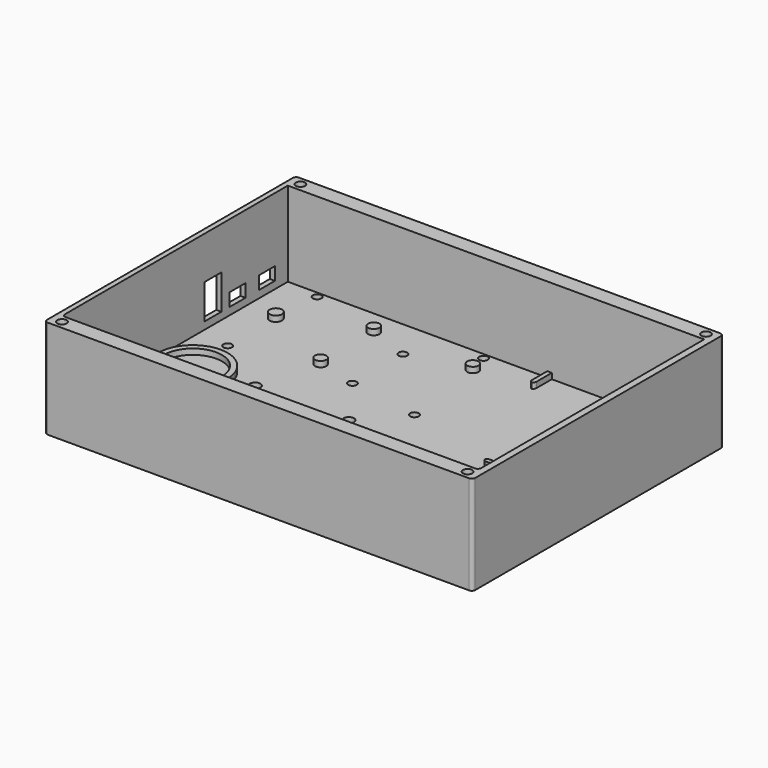
from build123d import *

# Parameters (mm, degrees)
F5_W         = 192.786
F5_H         = 141.3764
F7_DEPTH     = 44.45
F12_W        = 187.452
F12_H        = 127
F14_DEPTH    = 38.1
F4_R         = 15.621
F4_R_2       = 13.081
F13_W        = 2.032
F13_H        = 10.16
F13_W_2      = 10.16
F13_H_2      = 2.032
F15_DEPTH    = 8.89
F16_DEPTH    = 2.9972
F17_DEPTH    = 3.81
F10_R        = 2.3749
F18_DEPTH    = 25.4
F3_R         = 1.9304
F19_DEPTH    = 25.4
F11_R        = 2.54
F11_R_2      = 2.794
F20_DEPTH    = 8.89
F21_W        = 8.89
F21_H        = 5.842
F21_W_2      = 9.525
F21_H_2      = 15.621
F22_DEPTH    = 25.4
F23_R        = 2.0828
F24_DEPTH    = 4.318
F25_T1_DEPTH = 41.91
F25_T3_DEPTH = 52.07
F25_T5_DEPTH = 6.35


# Not quite as in the source:
# - a fillet or chamfer that OpenCascade refuses, or shapes differently, is made with other operations: its cross-section is extruded or revolved along the edge and cut away or added


with BuildPart() as f7:
    # F5 (on Top) → F7 (new body)
    with BuildSketch(Plane.XY):
        with Locations((-4.773771323, -23.1295908162)):
            Rectangle(F5_W, F5_H)
    extrude(amount=F7_DEPTH)

    # F12 (on face) → F14 (cut)
    with BuildSketch(Plane.XY.offset(44.45)):
        with Locations((-5.154771323, -23.1295908162)):
            Rectangle(F12_W, F12_H)
    extrude(amount=-F14_DEPTH, mode=Mode.SUBTRACT)

    # F4 (on Top) + F13 (on Top) → F15 (join)
    with BuildSketch(Plane.XY):
        with Locations((-81.989771323, -34.1785908162)):
            Circle(F4_R)
        with Locations((-81.989771323, -34.1785908162)):
            Circle(F4_R_2, mode=Mode.SUBTRACT)
    with BuildSketch(Plane.XY):
        with Locations((18.975228677, 35.2904091838)):
            Rectangle(F13_W, F13_H)
        with Locations((47.6495291469, -25.7965908162)):
            Rectangle(F13_W_2, F13_H_2)
    extrude(amount=F15_DEPTH)

    # F6 (on face) → F16 (cut)
    with BuildSketch(Plane.XY):
        Polygon((-81.6243755079, 34.3379091838), (-79.6079796927, 37.8304091838), (-81.6243755079, 41.3229091838), (-85.6571671382, 41.3229091838), (-87.6735629533, 37.8304091838), (-85.6571671382, 34.3379091838), align=None)
        Polygon((-6.6943755079, 34.3379091838), (-4.6779796927, 37.8304091838), (-6.6943755079, 41.3229091838), (-10.7271671382, 41.3229091838), (-12.7435629533, 37.8304091838), (-10.7271671382, 34.3379091838), align=None)
        Polygon((-30.8243755079, 19.0979091838), (-28.8079796927, 22.5904091838), (-30.8243755079, 26.0829091838), (-34.8571671382, 26.0829091838), (-36.8735629533, 22.5904091838), (-34.8571671382, 19.0979091838), align=None)
        Polygon((-82.8943755079, -14.4300908162), (-80.8779796927, -10.9375908162), (-82.8943755079, -7.4450908162), (-86.9271671382, -7.4450908162), (-88.9435629533, -10.9375908162), (-86.9271671382, -14.4300908162), align=None)
        Polygon((-30.8243755079, -9.3500908162), (-28.8079796927, -5.8575908162), (-30.8243755079, -2.3650908162), (-34.8571671382, -2.3650908162), (-36.8735629533, -5.8575908162), (-34.8571671382, -9.3500908162), align=None)
        Polygon((1.1796244921, -14.4300908162), (3.1960203073, -10.9375908162), (1.1796244921, -7.4450908162), (-2.8531671382, -7.4450908162), (-4.8695629533, -10.9375908162), (-2.8531671382, -14.4300908162), align=None)
    extrude(amount=F16_DEPTH, mode=Mode.SUBTRACT)

    # F9 (on Top) → F17 (cut)
    with BuildSketch(Plane.XY):
        Polygon((-55.7338586688, -33.239207965), (-53.0355544507, -28.565607965), (-55.7338586688, -23.892007965), (-61.130467105, -23.892007965), (-63.828771323, -28.565607965), (-61.130467105, -33.239207965), align=None)
        Polygon((-24.9998586688, -81.067407965), (-22.3015544507, -76.393807965), (-24.9998586688, -71.720207965), (-30.396467105, -71.720207965), (-33.094771323, -76.393807965), (-30.396467105, -81.067407965), align=None)
        Polygon((17.1641413312, -71.720207965), (14.4658371131, -71.720207965), (11.767532895, -71.720207965), (9.069228677, -76.393807965), (11.767532895, -81.067407965), (17.1641413312, -81.067407965), (19.8624455493, -76.393807965), align=None)
        Polygon((-10.8715544507, -28.565607965), (-13.5698586688, -23.892007965), (-18.966467105, -23.892007965), (-21.664771323, -28.565607965), (-18.966467105, -33.239207965), (-13.5698586688, -33.239207965), align=None)
    extrude(amount=F17_DEPTH, mode=Mode.SUBTRACT)

    # F10 (on Top) → F18 (cut)
    with BuildSketch(Plane.XY):
        with Locations((-58.4321628869, -28.565607965)):
            Circle(F10_R)
        with Locations((-27.6981628869, -76.393807965)):
            Circle(F10_R)
        with Locations((-16.2681628869, -28.565607965)):
            Circle(F10_R)
        with Locations((14.4658371131, -76.393807965)):
            Circle(F10_R)
    extrude(amount=F18_DEPTH, mode=Mode.SUBTRACT)

    # F3 (on Top) → F19 (cut)
    with BuildSketch(Plane.XY):
        with Locations((-84.910771323, -10.9375908162)):
            Circle(F3_R)
        with Locations((-32.840771323, -5.8575908162)):
            Circle(F3_R)
        with Locations((-32.840771323, 22.5904091838)):
            Circle(F3_R)
        with Locations((-8.710771323, 37.8304091838)):
            Circle(F3_R)
        with Locations((-83.640771323, 37.8304091838)):
            Circle(F3_R)
        with Locations((-0.836771323, -10.9375908162)):
            Circle(F3_R)
    extrude(amount=F19_DEPTH, mode=Mode.SUBTRACT)

    # F11 (on Top) → F20 (join)
    with BuildSketch(Plane.XY):
        with Locations((-6.1370921321, 28.5807047039)):
            Circle(F11_R)
        with Locations((-51.3140404916, 29.3099723562)):
            Circle(F11_R)
        with Locations((-50.6939233637, -1.3771463051)):
            Circle(F11_R)
        with Locations((-84.7697969953, 15.9851294398)):
            Circle(F11_R_2)
    extrude(amount=F20_DEPTH)

    # F21 (on face) → F22 (cut)
    with BuildSketch(Plane(origin=(-101.166771323, 0, 0), x_dir=(0, -1, 0), z_dir=(-1, 0, 0))):
        with Locations((-12.1256091838, 12.573)):
            Rectangle(F21_W, F21_H)
        with Locations((-28.6356091838, 12.573)):
            Rectangle(F21_W, F21_H)
        with Locations((1.7808908162, 17.4625)):
            Rectangle(F21_W_2, F21_H_2)
    extrude(amount=-F22_DEPTH, mode=Mode.SUBTRACT)

    # F23 (on face) → F24 (cut)
    with BuildSketch(Plane.XY.offset(44.45)):
        with Locations((-96.086771323, -90.2236908162)):
            Circle(F23_R)
        with Locations((86.539228677, -90.2236908162)):
            Circle(F23_R)
        with Locations((86.539228677, 43.9645091838)):
            Circle(F23_R)
        with Locations((-96.086771323, 43.9645091838)):
            Circle(F23_R)
    extrude(amount=-F24_DEPTH, mode=Mode.SUBTRACT)

    # F25: fillet of radius 1.524 on 12 edges, made by hand

    # F25_s2 → F25_t1 (join)
    with BuildSketch(Plane.XY.offset(2.54)):
        with BuildLine():
            ThreePointArc((-97.356771323, -86.6295908162), (-98.4344020576, -86.1832215507), (-98.880771323, -85.1055908162))
            Line((-98.880771323, -85.1055908162), (-98.880771323, -86.6295908162))
            Line((-98.880771323, -86.6295908162), (-97.356771323, -86.6295908162))
        make_face()
        with BuildLine():
            ThreePointArc((88.571228677, -85.1055908162), (88.1248594115, -86.1832215507), (87.047228677, -86.6295908162))
            Line((87.047228677, -86.6295908162), (88.571228677, -86.6295908162))
            Line((88.571228677, -86.6295908162), (88.571228677, -85.1055908162))
        make_face()
    extrude(amount=F25_T1_DEPTH)

    # F25_s4 → F25_t3 (cut)
    with BuildSketch(Plane.XY.offset(-3.81)):
        with BuildLine():
            ThreePointArc((-99.642771323, 47.5586091838), (-100.7204020576, 47.1122399184), (-101.166771323, 46.0346091838))
            Line((-101.166771323, 46.0346091838), (-101.166771323, 47.5586091838))
            Line((-101.166771323, 47.5586091838), (-99.642771323, 47.5586091838))
        make_face()
        with BuildLine():
            ThreePointArc((-101.166771323, -92.2937908162), (-100.7204020576, -93.3714215507), (-99.642771323, -93.8177908162))
            Line((-99.642771323, -93.8177908162), (-101.166771323, -93.8177908162))
            Line((-101.166771323, -93.8177908162), (-101.166771323, -92.2937908162))
        make_face()
        with BuildLine():
            ThreePointArc((91.619228677, -92.2937908162), (91.1728594115, -93.3714215507), (90.095228677, -93.8177908162))
            Line((90.095228677, -93.8177908162), (91.619228677, -93.8177908162))
            Line((91.619228677, -93.8177908162), (91.619228677, -92.2937908162))
        make_face()
        with BuildLine():
            ThreePointArc((90.095228677, 47.5586091838), (91.1728594115, 47.1122399184), (91.619228677, 46.0346091838))
            Line((91.619228677, 46.0346091838), (91.619228677, 47.5586091838))
            Line((91.619228677, 47.5586091838), (90.095228677, 47.5586091838))
        make_face()
    extrude(amount=F25_T3_DEPTH, mode=Mode.SUBTRACT)

    # F25_s6 → F25_t5 (cut)
    with BuildSketch(Plane.XY.offset(6.35)):
        with BuildLine():
            ThreePointArc((17.959228677, 31.7344091838), (18.4055979424, 30.6567784493), (19.483228677, 30.2104091838))
            Line((19.483228677, 30.2104091838), (17.959228677, 30.2104091838))
            Line((17.959228677, 30.2104091838), (17.959228677, 31.7344091838))
        make_face()
        with BuildLine():
            ThreePointArc((42.5695291469, -25.2885908162), (43.0158984124, -26.3662215507), (44.0935291469, -26.8125908162))
            Line((44.0935291469, -26.8125908162), (42.5695291469, -26.8125908162))
            Line((42.5695291469, -26.8125908162), (42.5695291469, -25.2885908162))
        make_face()
        with BuildLine():
            ThreePointArc((42.5695291469, -26.3045908162), (43.0158984124, -25.2269600816), (44.0935291469, -24.7805908162))
            Line((44.0935291469, -24.7805908162), (42.5695291469, -24.7805908162))
            Line((42.5695291469, -24.7805908162), (42.5695291469, -26.3045908162))
        make_face()
        with BuildLine():
            ThreePointArc((19.991228677, 31.7344091838), (19.5448594115, 30.6567784493), (18.467228677, 30.2104091838))
            Line((18.467228677, 30.2104091838), (19.991228677, 30.2104091838))
            Line((19.991228677, 30.2104091838), (19.991228677, 31.7344091838))
        make_face()
        with BuildLine():
            ThreePointArc((51.2055291469, -26.8125908162), (52.2831598814, -26.3662215507), (52.7295291469, -25.2885908162))
            Line((52.7295291469, -25.2885908162), (52.7295291469, -26.8125908162))
            Line((52.7295291469, -26.8125908162), (51.2055291469, -26.8125908162))
        make_face()
        with BuildLine():
            ThreePointArc((51.2055291469, -24.7805908162), (52.2831598814, -25.2269600816), (52.7295291469, -26.3045908162))
            Line((52.7295291469, -26.3045908162), (52.7295291469, -24.7805908162))
            Line((52.7295291469, -24.7805908162), (51.2055291469, -24.7805908162))
        make_face()
    extrude(amount=F25_T5_DEPTH, mode=Mode.SUBTRACT)


solid = f7.part
